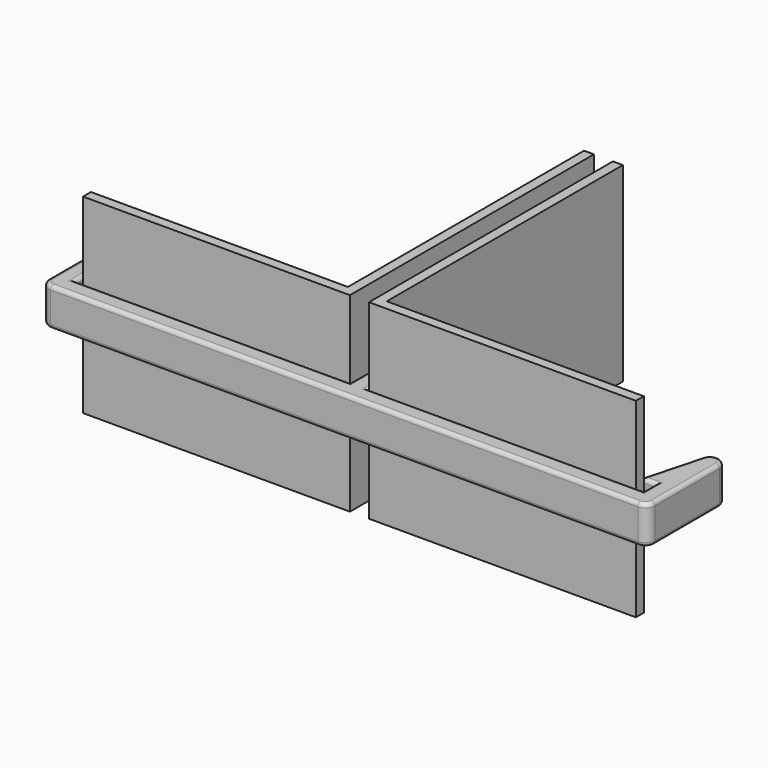
from build123d import *

# Parameters (mm, degrees)
F2_DEPTH     = 2.5
F4_R         = 1.25
F5_DEPTH     = 2.5
F6_R         = 1
F7_R         = 0.5
F8_T1_DEPTH  = 5
F8_T4_ANGLE  = 90
F8_T6_ANGLE  = 90
F8_T8_ANGLE  = 90
F8_T10_ANGLE = 90
F8_T12_ANGLE = 165
F8_T14_ANGLE = 165
F8_T16_ANGLE = 165
F8_T18_ANGLE = 165
F8_T20_ANGLE = 90
F8_T22_ANGLE = 90
F8_T24_ANGLE = 90
F8_T26_ANGLE = 90
F0_W         = 8
F0_H         = 1.3
F0_W_2       = 4
F9_DEPTH     = 12.5


# Not quite as in the source:
# - a fillet or chamfer that OpenCascade refuses, or shapes differently, is made with other operations: its cross-section is extruded or revolved along the edge and cut away or added


with BuildPart() as f2:
    # F1 (on Top) → F2 (new body, symmetric)
    with BuildSketch(Plane.XY):
        Polygon((-37.25, 0), (-37.25, 2), (-35.25, 2), (-39.75, 18.7942286341), (-39.75, -2.5), (0, -2.5), (0, 30), (-1.25, 30), (-1.25, 0), align=None)
    extrude(amount=F2_DEPTH, both=True)

    # F3: F2 across plane


with BuildPart() as f2_1:
    add(f2.part)
    add(f2.part.mirror(Plane.YZ))

    # F4 (on face) → F5 (join)
    with BuildSketch(Plane(origin=(0, 0, 0), x_dir=(-1, 0, 0), z_dir=(0, 1, 0))):
        with Locations((26.25, 0)):
            Circle(F4_R)
    extrude(amount=F5_DEPTH)

    # F6
    f6_edges = [f2_1.edges().sort_by_distance(p)[0] for p in [
        (-25, 2.5, 0),
    ]]
    fillet(f6_edges, radius=F6_R)

    # F7
    f7_edges = [f2_1.edges().sort_by_distance(p)[0] for p in [
        (-37.25, 1, -2.5),
        (-36.25, 2, -2.5),
        (-37.5, 10.397114, -2.5),
        (-39.75, 8.147114, -2.5),
        (0, -2.5, -2.5),
        (39.75, 8.147114, -2.5),
        (37.5, 10.397114, -2.5),
        (36.25, 2, -2.5),
        (37.25, 1, -2.5),
        (19.25, 0, -2.5),
        (1.25, 15, -2.5),
        (0, 30, -2.5),
        (-1.25, 15, -2.5),
        (-19.25, 0, -2.5),
        (-37.25, 1, 2.5),
        (-36.25, 2, 2.5),
        (-37.5, 10.397114, 2.5),
        (-39.75, 8.147114, 2.5),
        (0, -2.5, 2.5),
        (39.75, 8.147114, 2.5),
        (37.5, 10.397114, 2.5),
        (36.25, 2, 2.5),
        (37.25, 1, 2.5),
        (19.25, 0, 2.5),
        (1.25, 15, 2.5),
        (0, 30, 2.5),
        (-1.25, 15, 2.5),
        (-19.25, 0, 2.5),
    ]]
    fillet(f7_edges, radius=F7_R)

    # F8: fillet of radius 1.25 on 6 edges, made by hand

    # F8_s2 → F8_t1 (cut)
    with BuildSketch(Plane.XY.offset(-2.5)):
        with BuildLine():
            ThreePointArc((0, 30), (0.8838834765, 29.6338834765), (1.25, 28.75))
            Line((1.25, 28.75), (1.25, 30))
            Line((1.25, 30), (0, 30))
        make_face()
        with BuildLine():
            ThreePointArc((-1.25, 28.75), (-0.8838834765, 29.6338834765), (0, 30))
            Line((0, 30), (-1.25, 30))
            Line((-1.25, 30), (-1.25, 28.75))
        make_face()
        with BuildLine():
            ThreePointArc((-37.2925927171, 9.6230597995), (-38.6631577403, 10.5388420699), (-39.75, 9.2995359932))
            Line((-39.75, 9.2995359932), (-39.75, 18.7942286341))
            Line((-39.75, 18.7942286341), (-37.2925927171, 9.6230597995))
        make_face()
        with BuildLine():
            ThreePointArc((39.75, 9.2995359932), (38.6631577403, 10.5388420699), (37.2925927171, 9.6230597995))
            Line((37.2925927171, 9.6230597995), (39.75, 18.7942286341))
            Line((39.75, 18.7942286341), (39.75, 9.2995359932))
        make_face()
        with BuildLine():
            ThreePointArc((38.5, -2.5), (39.3838834765, -2.1338834765), (39.75, -1.25))
            Line((39.75, -1.25), (39.75, -2.5))
            Line((39.75, -2.5), (38.5, -2.5))
        make_face()
        with BuildLine():
            ThreePointArc((-39.75, -1.25), (-39.3838834765, -2.1338834765), (-38.5, -2.5))
            Line((-38.5, -2.5), (-39.75, -2.5))
            Line((-39.75, -2.5), (-39.75, -1.25))
        make_face()
    extrude(amount=F8_T1_DEPTH, mode=Mode.SUBTRACT)

    # F8_s3 → F8_t4 (revolve, cut)
    with BuildSketch(Plane.YZ.offset(-38.5)):
        with BuildLine():
            ThreePointArc((-2, -2.5), (-2.3535533906, -2.3535533906), (-2.5, -2))
            Line((-2.5, -2), (-2.5, -2.5))
            Line((-2.5, -2.5), (-2, -2.5))
        make_face()
    revolve(axis=Axis((-38.5, -1.25, -2.5), (0, 0, -1)), revolution_arc=F8_T4_ANGLE, mode=Mode.SUBTRACT)

    # F8_s5 → F8_t6 (revolve, cut)
    with BuildSketch(Plane.XZ.offset(1.25)):
        with BuildLine():
            ThreePointArc((-39.25, 2.5), (-39.6035533906, 2.3535533906), (-39.75, 2))
            Line((-39.75, 2), (-39.75, 2.5))
            Line((-39.75, 2.5), (-39.25, 2.5))
        make_face()
    revolve(axis=Axis((-38.5, -1.25, 2.5), (0, 0, 1)), revolution_arc=F8_T6_ANGLE, mode=Mode.SUBTRACT)

    # F8_s7 → F8_t8 (revolve, cut)
    with BuildSketch(Plane.XZ.offset(1.25)):
        with BuildLine():
            ThreePointArc((39.25, -2.5), (39.6035533906, -2.3535533906), (39.75, -2))
            Line((39.75, -2), (39.75, -2.5))
            Line((39.75, -2.5), (39.25, -2.5))
        make_face()
    revolve(axis=Axis((38.5, -1.25, -2.5), (0, 0, -1)), revolution_arc=F8_T8_ANGLE, mode=Mode.SUBTRACT)

    # F8_s9 → F8_t10 (revolve, cut)
    with BuildSketch(Plane.YZ.offset(38.5)):
        with BuildLine():
            ThreePointArc((-2, 2.5), (-2.3535533906, 2.3535533906), (-2.5, 2))
            Line((-2.5, 2), (-2.5, 2.5))
            Line((-2.5, 2.5), (-2, 2.5))
        make_face()
    revolve(axis=Axis((38.5, -1.25, 2.5), (0, 0, 1)), revolution_arc=F8_T10_ANGLE, mode=Mode.SUBTRACT)

    # F8_s11 → F8_t12 (revolve, cut)
    with BuildSketch(Plane(origin=(4.9038949754, 18.3015852033, 0), x_dir=(0, 0, 1), z_dir=(-0.2588190451, -0.9659258263, 0))):
        with BuildLine():
            ThreePointArc((-2.5, -34.0312472865), (-2.3535533906, -33.6776938959), (-2, -33.5312472865))
            Line((-2, -33.5312472865), (-2.5, -33.5312472865))
            Line((-2.5, -33.5312472865), (-2.5, -34.0312472865))
        make_face()
    revolve(axis=Axis((38.5, 9.2995359932, -2.5), (0, 0, -1)), revolution_arc=F8_T12_ANGLE, mode=Mode.SUBTRACT)

    # F8_s13 → F8_t14 (revolve, cut)
    with BuildSketch(Plane.XZ.offset(-9.2995359932)):
        with BuildLine():
            ThreePointArc((39.25, 2.5), (39.6035533906, 2.3535533906), (39.75, 2))
            Line((39.75, 2), (39.75, 2.5))
            Line((39.75, 2.5), (39.25, 2.5))
        make_face()
    revolve(axis=Axis((38.5, 9.2995359932, 2.5), (0, 0, 1)), revolution_arc=F8_T14_ANGLE, mode=Mode.SUBTRACT)

    # F8_s15 → F8_t16 (revolve, cut)
    with BuildSketch(Plane.XZ.offset(-9.2995359932)):
        with BuildLine():
            ThreePointArc((-39.25, -2.5), (-39.6035533906, -2.3535533906), (-39.75, -2))
            Line((-39.75, -2), (-39.75, -2.5))
            Line((-39.75, -2.5), (-39.25, -2.5))
        make_face()
    revolve(axis=Axis((-38.5, 9.2995359932, -2.5), (0, 0, -1)), revolution_arc=F8_T16_ANGLE, mode=Mode.SUBTRACT)

    # F8_s17 → F8_t18 (revolve, cut)
    with BuildSketch(Plane(origin=(-4.9038949754, 18.3015852033, 0), x_dir=(0, 0, 1), z_dir=(0.2588190451, -0.9659258263, 0))):
        with BuildLine():
            ThreePointArc((2.5, 34.0312472865), (2.3535533906, 33.6776938959), (2, 33.5312472865))
            Line((2, 33.5312472865), (2.5, 33.5312472865))
            Line((2.5, 33.5312472865), (2.5, 34.0312472865))
        make_face()
    revolve(axis=Axis((-38.5, 9.2995359932, 2.5), (0, 0, 1)), revolution_arc=F8_T18_ANGLE, mode=Mode.SUBTRACT)

    # F8_s19 → F8_t20 (revolve, cut)
    with BuildSketch(Plane.YZ):
        with BuildLine():
            ThreePointArc((29.5, 2.5), (29.8535533906, 2.3535533906), (30, 2))
            Line((30, 2), (30, 2.5))
            Line((30, 2.5), (29.5, 2.5))
        make_face()
    revolve(axis=Axis((0, 28.75, 2.5), (0, 0, 1)), revolution_arc=F8_T20_ANGLE, mode=Mode.SUBTRACT)

    # F8_s21 → F8_t22 (revolve, cut)
    with BuildSketch(Plane.XZ.offset(-28.75)):
        with BuildLine():
            ThreePointArc((-0.75, -2.5), (-1.1035533906, -2.3535533906), (-1.25, -2))
            Line((-1.25, -2), (-1.25, -2.5))
            Line((-1.25, -2.5), (-0.75, -2.5))
        make_face()
    revolve(axis=Axis((0, 28.75, -2.5), (0, 0, -1)), revolution_arc=F8_T22_ANGLE, mode=Mode.SUBTRACT)

    # F8_s23 → F8_t24 (revolve, cut)
    with BuildSketch(Plane.XZ.offset(-28.75)):
        with BuildLine():
            ThreePointArc((0.75, 2.5), (1.1035533906, 2.3535533906), (1.25, 2))
            Line((1.25, 2), (1.25, 2.5))
            Line((1.25, 2.5), (0.75, 2.5))
        make_face()
    revolve(axis=Axis((0, 28.75, 2.5), (0, 0, 1)), revolution_arc=F8_T24_ANGLE, mode=Mode.SUBTRACT)

    # F8_s25 → F8_t26 (revolve, cut)
    with BuildSketch(Plane.YZ):
        with BuildLine():
            ThreePointArc((29.5, -2.5), (29.8535533906, -2.3535533906), (30, -2))
            Line((30, -2), (30, -2.5))
            Line((30, -2.5), (29.5, -2.5))
        make_face()
    revolve(axis=Axis((0, 28.75, -2.5), (0, 0, -1)), revolution_arc=F8_T26_ANGLE, mode=Mode.SUBTRACT)


with BuildPart() as f9:
    # F0 (on Top) → F9 (new body, symmetric)
    with BuildSketch(Plane.XY):
        Polygon((-24.25, 0), (-1.25, 0), (-1.25, 40), (-2.55, 40), (-2.55, 1.3), (-24.25, 1.3), align=None)
        with Locations((-32.25, 0.65)):
            Rectangle(F0_W, F0_H)
        with Locations((-26.25, 0.65)):
            Rectangle(F0_W_2, F0_H)
    extrude(amount=F9_DEPTH, both=True)


with BuildPart() as f10_1:
    # F10: instance of F9
    add(f9.part.mirror(Plane.YZ))


solid = Compound([f2_1.part, f9.part, f10_1.part])
